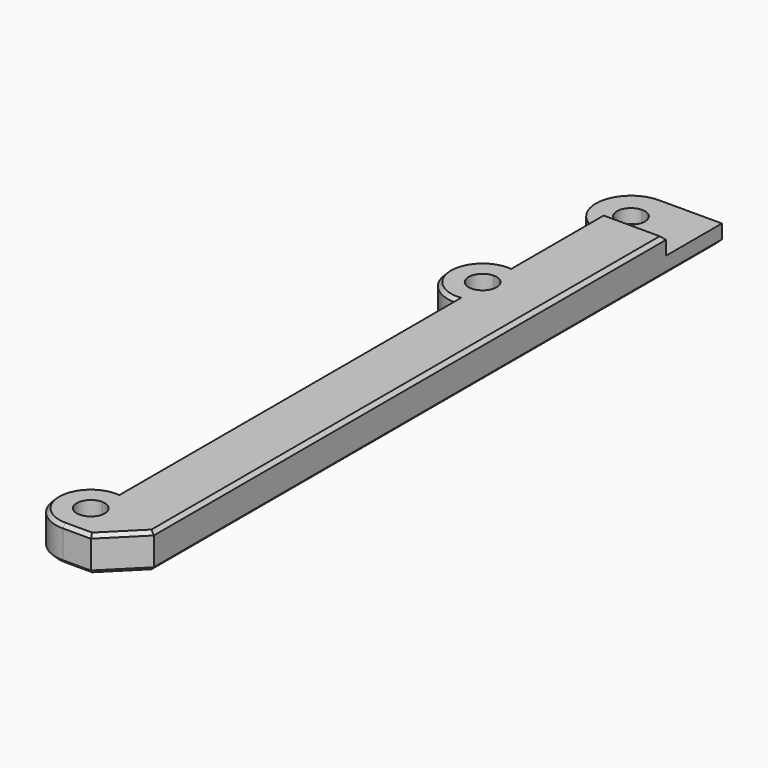
from build123d import *

# Parameters (mm, degrees)
F1_DEPTH = 5
F3_DEPTH = 2.5
F4_SIZE  = 5
F5_SIZE  = 0.5


with BuildPart() as f1:
    # F0 (on Top) → F1 (new body)
    with BuildSketch(Plane.XY):
        with BuildLine():
            Line((-9, 0), (0, 0))
            Line((0, 0), (0, 106.5))
            Line((0, 106.5), (-9, 106.5))
            Line((-9, 106.5), (-9, 103.5))
            ThreePointArc((-9, 103.5), (-7.5857864376, 102.9142135624), (-7, 101.5))
            ThreePointArc((-7, 101.5), (-7.5857864376, 100.0857864376), (-9, 99.5))
            Line((-9, 99.5), (-9, 96.5))
            Line((-9, 96.5), (-9, 80))
            Line((-9, 80), (-9, 77))
            ThreePointArc((-9, 77), (-7.5857864376, 76.4142135624), (-7, 75))
            ThreePointArc((-7, 75), (-7.5857864376, 73.5857864376), (-9, 73))
            Line((-9, 73), (-9, 70))
            Line((-9, 70), (-9, 10))
            Line((-9, 10), (-9, 7))
            ThreePointArc((-9, 7), (-7.5857864376, 6.4142135624), (-7, 5))
            ThreePointArc((-7, 5), (-7.5857864376, 3.5857864376), (-9, 3))
            Line((-9, 3), (-9, 0))
        make_face()
        with BuildLine():
            ThreePointArc((-9, 10), (-14, 5), (-9, 0))
            Line((-9, 0), (-9, 3))
            ThreePointArc((-9, 3), (-11, 5), (-9, 7))
            Line((-9, 7), (-9, 10))
        make_face()
        with BuildLine():
            Line((-9, 103.5), (-9, 106.5))
            ThreePointArc((-9, 106.5), (-14, 101.5), (-9, 96.5))
            Line((-9, 96.5), (-9, 99.5))
            ThreePointArc((-9, 99.5), (-11, 101.5), (-9, 103.5))
        make_face()
        with BuildLine():
            ThreePointArc((-9, 80), (-14, 75), (-9, 70))
            Line((-9, 70), (-9, 73))
            ThreePointArc((-9, 73), (-11, 75), (-9, 77))
            Line((-9, 77), (-9, 80))
        make_face()
    extrude(amount=F1_DEPTH)

    # F2 (on face) → F3 (cut)
    with BuildSketch(Plane.XY.offset(5)):
        with BuildLine():
            ThreePointArc((-9, 106.5), (-14, 101.5), (-9, 96.5))
            Line((-9, 96.5), (0, 96.5))
            Line((0, 96.5), (0, 106.5))
            Line((0, 106.5), (-9, 106.5))
        make_face()
    extrude(amount=-F3_DEPTH, mode=Mode.SUBTRACT)

    # F4
    f4_edges = [f1.edges().sort_by_distance(p)[0] for p in [
        (0, 0, 2.5),
    ]]
    chamfer(f4_edges, length=F4_SIZE)

    # F5
    f5_edges = [f1.edges().sort_by_distance(p)[0] for p in [
        (-7, 0, 0),
        (-2.5, 2.5, 0),
        (-14, 5, 0),
        (0, 55.75, 0),
        (-9, 40, 0),
        (-4.5, 106.5, 0),
        (-14, 75, 0),
        (-14, 101.5, 0),
        (-9, 88.25, 0),
        (-9, 77, 0),
        (-9, 103.5, 0),
        (-11, 5, 0),
        (-4.5, 96.5, 5),
        (0, 50.75, 5),
        (-9, 88.25, 5),
        (-14, 75, 5),
        (-2.5, 2.5, 5),
        (-7, 0, 5),
        (-14, 5, 5),
        (-9, 40, 5),
    ]]
    chamfer(f5_edges, length=F5_SIZE)


solid = f1.part
